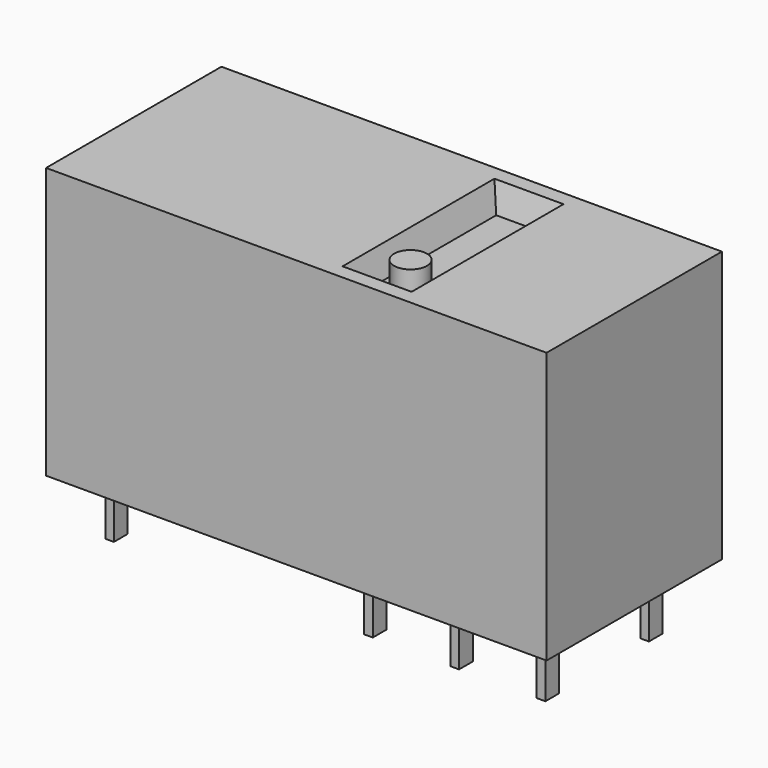
from build123d import *

# Parameters (mm, degrees)
F0_W     = 12.7
F0_H     = 15.7
F1_DEPTH = 14.5
F2_W     = 0.5
F2_H     = 1
F3_DEPTH = 3.5
F4_W     = 4
F4_H     = 11
F4_R     = 0.9543570249
F5_DEPTH = 1.5
F6_SIZE2 = 1.49999
F6_SIZE  = 0.49999


# Not quite as in the source:
# - a fillet or chamfer is up to 0.001 mm smaller than in the source, because OpenCascade refuses the exact size


with BuildPart() as f1:
    # F0 (on Right) → F1 (new body, symmetric)
    with BuildSketch(Plane.YZ):
        with Locations((0, 7.85)):
            Rectangle(F0_W, F0_H)
    extrude(amount=F1_DEPTH, both=True)

    # F2 (on Top) → F3 (join)
    with BuildSketch(Plane.XY):
        with Locations((-12.5, 3.75)):
            Rectangle(F2_W, F2_H)
        with Locations((2.5, 3.75)):
            Rectangle(F2_W, F2_H)
        with Locations((7.5, 3.75)):
            Rectangle(F2_W, F2_H)
        with Locations((12.5, 3.75)):
            Rectangle(F2_W, F2_H)
        with Locations((2.5, -3.75)):
            Rectangle(F2_W, F2_H)
        with Locations((7.5, -3.75)):
            Rectangle(F2_W, F2_H)
        with Locations((12.5, -3.75)):
            Rectangle(F2_W, F2_H)
        with Locations((-12.5, -3.75)):
            Rectangle(F2_W, F2_H)
    extrude(amount=-F3_DEPTH)

    # F4 (on face) → F5 (cut)
    with BuildSketch(Plane.XY.offset(15.7)):
        with Locations((4, 0)):
            Rectangle(F4_W, F4_H)
        with Locations((4, -3.076559362)):
            Circle(F4_R, mode=Mode.SUBTRACT)
    extrude(amount=-F5_DEPTH, mode=Mode.SUBTRACT)

    # F6 (size 0.5 and 1.5 in the source; OpenCascade refuses exactly that, so slightly less here)
    f6_edges = [f1.edges().sort_by_distance(p)[0] for p in [
        (2, 0, 14.2),
        (4, 5.5, 14.2),
        (6, 0, 14.2),
        (4, -5.5, 14.2),
    ]]
    f6_side = f1.faces().sort_by_distance((4, 0.213987, 14.2))[0]
    chamfer(f6_edges, length=F6_SIZE, length2=F6_SIZE2, reference=f6_side)


solid = f1.part
